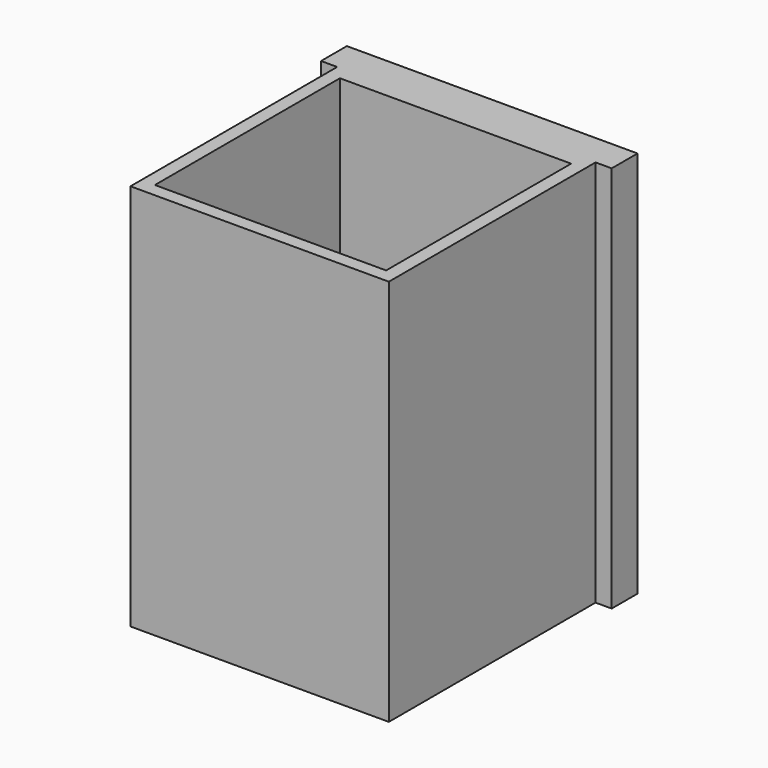
from build123d import *

# Parameters (mm, degrees)
F0_W     = 57.15
F0_H     = 76.2
F2_DEPTH = 6.35
F1_W     = 50.8
F1_H     = 50.8
F1_W_2   = 45.466
F1_H_2   = 45.466
F3_DEPTH = 38.1
F4_START = -33.655
F4_DEPTH = 4.445


# Not quite as in the source:
# - a feature names something its author has since deleted; it is built from what else it names


with BuildPart() as f2:
    # F0 (on Front) → F2 (new body)
    with BuildSketch(Plane.XZ):
        Rectangle(F0_W, F0_H)
    extrude(amount=-F2_DEPTH)

    # F1 (on Top) → F3 (join, symmetric)
    with BuildSketch(Plane.XY):
        with Locations((0, -25.4)):
            Rectangle(F1_W, F1_H)
        with Locations((0, -25.4)):
            Rectangle(F1_W_2, F1_H_2, mode=Mode.SUBTRACT)
    extrude(amount=F3_DEPTH, both=True)

    # F1 (on Top) → F4 (join)
    with BuildSketch(Plane.XY.offset(F4_START)):
        with Locations((0, -25.4)):
            Rectangle(F1_W_2, F1_H_2)
    extrude(amount=-F4_DEPTH)


solid = f2.part
